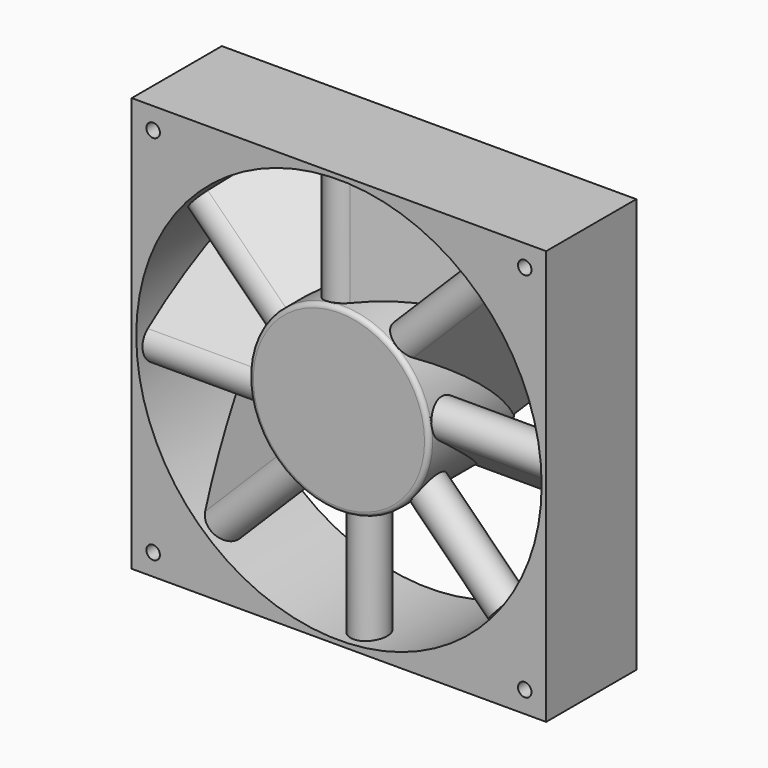
from build123d import *

# Parameters (mm, degrees)
F0_W     = 92
F0_H     = 92
F0_R     = 1.5
F0_R_2   = 45
F1_DEPTH = 25
F3_DEPTH = 50
F4_COUNT = 8
F5_R     = 20
F6_DEPTH = 25
F7_W     = 120
F7_H     = 120
F7_R     = 44.5
F8_DEPTH = 25.0010001
F9_R     = 0.99999


# Not quite as in the source:
# - a fillet or chamfer is up to 0.001 mm smaller than in the source, because OpenCascade refuses the exact size


with BuildPart() as f1:
    # F0 (on Front) → F1 (new body)
    with BuildSketch(Plane.XZ):
        Rectangle(F0_W, F0_H)
        with Locations((-41.25, -41.25)):
            Circle(F0_R, mode=Mode.SUBTRACT)
        with Locations((41.25, -41.25)):
            Circle(F0_R, mode=Mode.SUBTRACT)
        with Locations((-41.25, 41.25)):
            Circle(F0_R, mode=Mode.SUBTRACT)
        Circle(F0_R_2, mode=Mode.SUBTRACT)
        with Locations((41.25, 41.25)):
            Circle(F0_R, mode=Mode.SUBTRACT)
    extrude(amount=-F1_DEPTH)


with BuildPart() as f3:
    # F2 (on Right) → F3 (new body)
    with BuildSketch(Plane.YZ):
        with BuildLine():
            ThreePointArc((8.2495088034, 5.0992883494), (2.2165993594, 5.6395071005), (2.5659984731, -0.4074551879))
            Line((2.5659984731, -0.4074551879), (24, -16.8431419879))
            Line((24, -16.8431419879), (8.2495088034, 5.0992883494))
        make_face()
    extrude(amount=F3_DEPTH)


with BuildPart() as f4_1:
    # F4: instance of F3
    add(f3.part.rotate(Axis((0, -8.8478960097, 0), (0, -1, 0)), 1 * 360 / F4_COUNT))


with BuildPart() as f4_2:
    # F4: instance of F3
    add(f3.part.rotate(Axis((0, -8.8478960097, 0), (0, -1, 0)), 2 * 360 / F4_COUNT))


with BuildPart() as f4_3:
    # F4: instance of F3
    add(f3.part.rotate(Axis((0, -8.8478960097, 0), (0, -1, 0)), 3 * 360 / F4_COUNT))


with BuildPart() as f4_4:
    # F4: instance of F3
    add(f3.part.rotate(Axis((0, -8.8478960097, 0), (0, -1, 0)), 4 * 360 / F4_COUNT))


with BuildPart() as f4_5:
    # F4: instance of F3
    add(f3.part.rotate(Axis((0, -8.8478960097, 0), (0, -1, 0)), 5 * 360 / F4_COUNT))


with BuildPart() as f4_6:
    # F4: instance of F3
    add(f3.part.rotate(Axis((0, -8.8478960097, 0), (0, -1, 0)), 6 * 360 / F4_COUNT))


with BuildPart() as f4_7:
    # F4: instance of F3
    add(f3.part.rotate(Axis((0, -8.8478960097, 0), (0, -1, 0)), 7 * 360 / F4_COUNT))


with BuildPart() as f3_1:
    add(f3.part)

    add(f4_1.part)  # F6 merges F4_1

    add(f4_2.part)  # F6 merges F4_2

    add(f4_3.part)  # F6 merges F4_3

    add(f4_4.part)  # F6 merges F4_4

    add(f4_5.part)  # F6 merges F4_5

    add(f4_6.part)  # F6 merges F4_6

    add(f4_7.part)  # F6 merges F4_7
    # F5 (on Front) → F6 (join)
    with BuildSketch(Plane.XZ):
        Circle(F5_R)
    extrude(amount=-F6_DEPTH)

    # F7 (on Front) → F8 (cut, through all)
    with BuildSketch(Plane.XZ):
        Rectangle(F7_W, F7_H)
        Circle(F7_R, mode=Mode.SUBTRACT)
    extrude(amount=-F8_DEPTH, mode=Mode.SUBTRACT)

    # F9 (radius 1 in the source; OpenCascade refuses exactly that, so slightly less here)
    f9_edges = [f3_1.edges().sort_by_distance(p)[0] for p in [
        (-20, 0, 0),
        (-20, 25, 0),
    ]]
    fillet(f9_edges, radius=F9_R)


solid = Compound([f1.part, f3_1.part])
